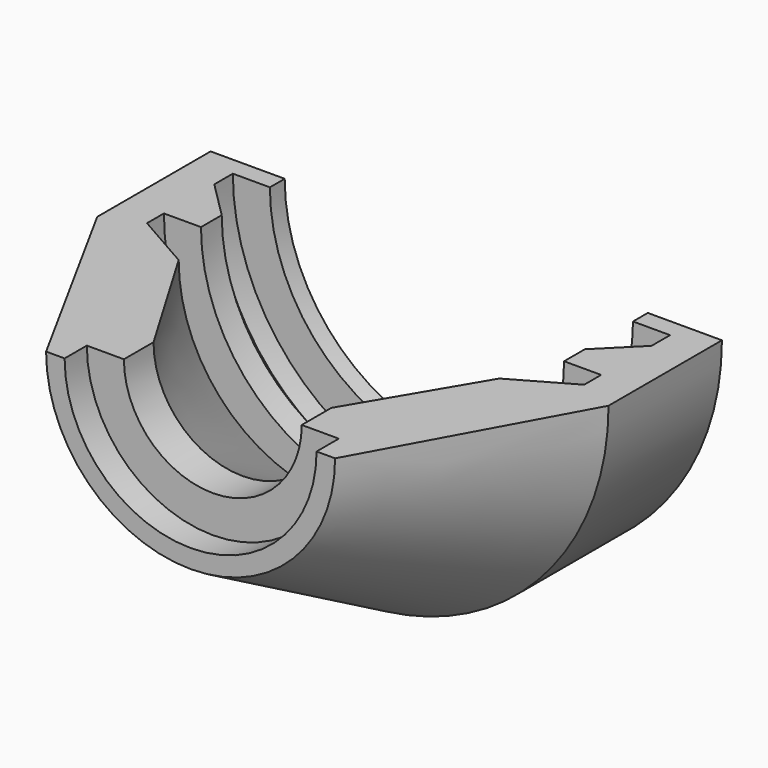
from build123d import *

# Parameters (mm, degrees)
F1_ANGLE    = 180
F2_T4_ANGLE = 248.1806251609
F2_S5_R     = 11.8
F2_T6_DEPTH = 17
F3_T4_ANGLE = 247.7679532438
F3_S5_R     = 11.8
F3_T6_DEPTH = 17


# Not quite as in the source:
# - a fillet or chamfer that OpenCascade refuses, or shapes differently, is made with other operations: its cross-section is extruded or revolved along the edge and cut away or added


with BuildPart() as f1:
    # F0 (on Top) → F1 (revolve)
    with BuildSketch(Plane.XY):
        Polygon((-11.8, 5.65), (-11.8, 6.65), (-13.8, 6.65), (-13.8, 0), (-7.8, -10.95), (-6.8, -10.95), (-6.8, -9.45), (-4.8, -9.45), (-4.8, -7.45), (-9.8, 1), (-11.8, 1), (-11.8, 2), (-9.8, 2), (-9.8, 5.65), align=None)
        Polygon((-13.8, 6.65), (-11.8, 6.65), (-9.8, 6.65), (-9.8, 7.65), (-13.8, 7.65), align=None)
    revolve(axis=Axis((0, 0, 0), (0, -1, 0)), revolution_arc=F1_ANGLE)

    # F2: chamfer of 2.25 on 1 edges, made by hand


with BuildPart() as f2_tool2:
    # F2_s3 → F2_t4 (revolve)
    with BuildSketch(Plane(origin=(0, 0, 0), x_dir=(0, 1, 0), z_dir=(0.5604989803, 0, 0.8281551142))):
        Polygon((-0.9364000214, 8.6542011708), (1, 12.05), (1, 9.8), align=None)
    revolve(axis=Axis((0, 1, 0), (0, -1, 0)), revolution_arc=F2_T4_ANGLE)

    # F2_s5 → F2_t6 (intersect, symmetric)
    with BuildSketch(Plane.XZ):
        Circle(F2_S5_R)
    extrude(amount=F2_T6_DEPTH, both=True, mode=Mode.INTERSECT)


with BuildPart() as f1_1:
    add(f1.part)

    # F2_t1: cut F2_tool2
    add(f2_tool2.part, mode=Mode.SUBTRACT)

    # F3: chamfer of 2.25 on 1 edges, made by hand


with BuildPart() as f3_tool2:
    # F3_s3 → F3_t4 (revolve)
    with BuildSketch(Plane(origin=(0, 0, 0), x_dir=(0, 1, 0), z_dir=(0.5575129654, 0, 0.830168232))):
        Polygon((5.65, 12.05), (3.4, 9.8), (5.65, 9.8), align=None)
    revolve(axis=Axis((0, 5.65, 0), (0, -1, 0)), revolution_arc=F3_T4_ANGLE)

    # F3_s5 → F3_t6 (intersect, symmetric)
    with BuildSketch(Plane.XZ.offset(-4.5)):
        Circle(F3_S5_R)
    extrude(amount=F3_T6_DEPTH, both=True, mode=Mode.INTERSECT)


with BuildPart() as f1_2:
    add(f1_1.part)

    # F3_t1: cut F3_tool2
    add(f3_tool2.part, mode=Mode.SUBTRACT)


solid = f1_2.part
